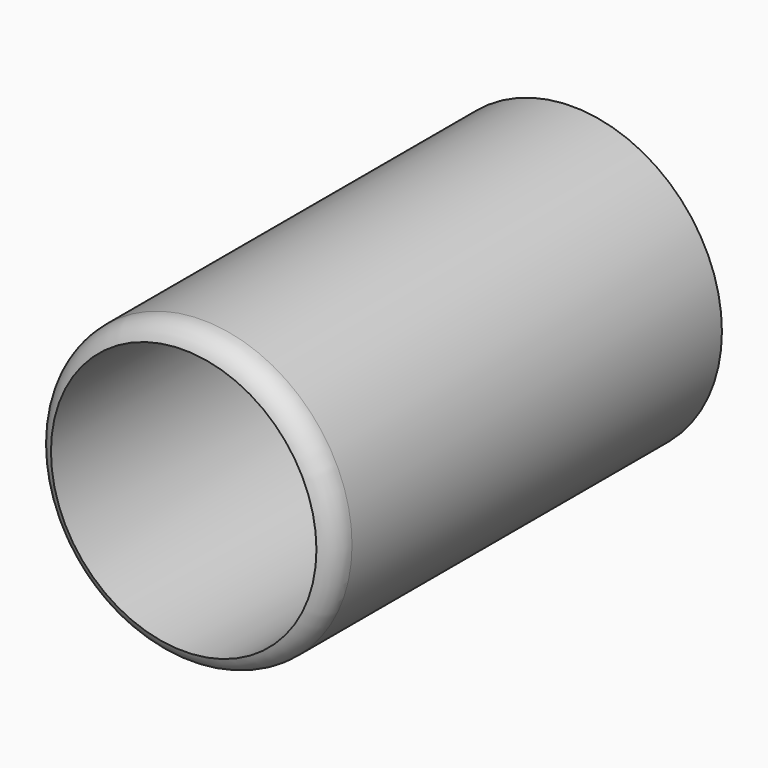
from build123d import *

# Parameters (mm, degrees)
F0_R     = 38.1
F0_R_2   = 33.8298969846
F1_DEPTH = 123.825
F2_DEPTH = 9.525
F4_DEPTH = 12.7
F5_R     = 35.7824148946
F6_DEPTH = 25.4


# Not quite as in the source:
# - a fillet or chamfer that OpenCascade refuses, or shapes differently, is made with other operations: its cross-section is extruded or revolved along the edge and cut away or added


with BuildPart() as f1:
    # F0 (on Front) → F1 (new body)
    with BuildSketch(Plane.XZ):
        Circle(F0_R)
        Circle(F0_R_2, mode=Mode.SUBTRACT)
    extrude(amount=F1_DEPTH)

    # F0 (on Front) → F2 (join)
    with BuildSketch(Plane.XZ):
        Circle(F0_R)
        Circle(F0_R_2, mode=Mode.SUBTRACT)
    extrude(amount=F2_DEPTH)

    # F3: fillet of radius 6.35 on 1 edges, made by hand

    # F3_s1 → F3_t2 (revolve, cut)
    with BuildSketch(Plane.XY):
        with BuildLine():
            ThreePointArc((38.1, -117.8252892959), (36.923482669, -121.5073508209), (33.8298969846, -123.825))
            Line((33.8298969846, -123.825), (38.1, -123.825))
            Line((38.1, -123.825), (38.1, -117.8252892959))
        make_face()
    revolve(axis=Axis((0, -123.825, 0), (0, -1, 0)), mode=Mode.SUBTRACT)

    # F0 (on Front) → F4 (join)
    with BuildSketch(Plane.XZ):
        Circle(F0_R)
        Circle(F0_R_2, mode=Mode.SUBTRACT)
    extrude(amount=F4_DEPTH)

    # F5 (on Front) → F6 (join)
    with BuildSketch(Plane.XZ):
        Circle(F5_R)
    extrude(amount=F6_DEPTH)


solid = f1.part
